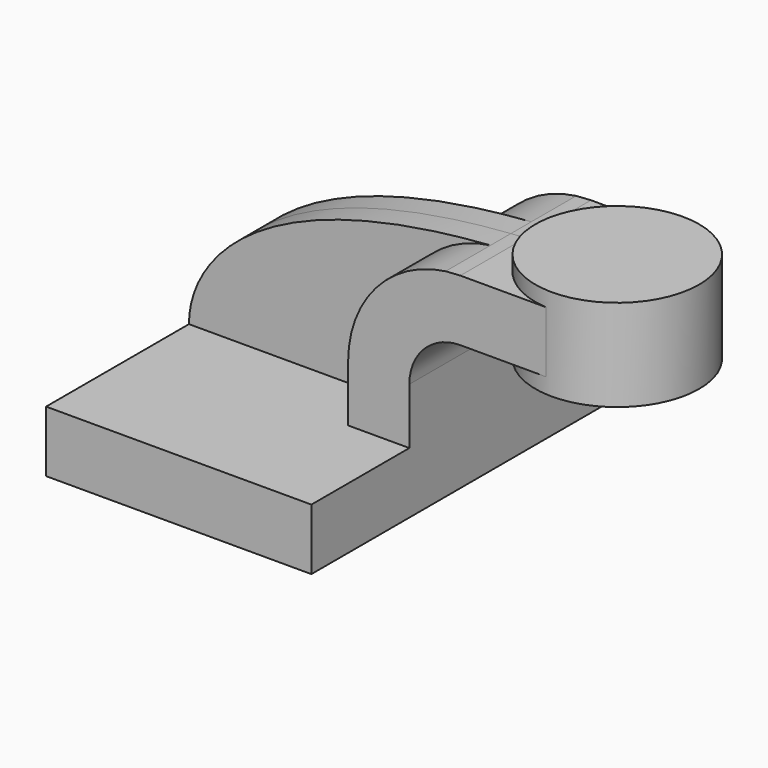
from build123d import *

# Parameters (mm, degrees)
F1_DEPTH = 63.5
F0_W     = 25.3298562567
F0_H     = 19.05
F2_DEPTH = 25.4
F3_DEPTH = 7.9375


with BuildPart() as f1:
    # F0 (on Front) → F1 (new body, symmetric)
    with BuildSketch(Plane.XZ):
        Polygon((-41.275, 9.525), (-41.275, -9.525), (41.275, -9.525), (41.275, 9.525), (22.225, 9.525), align=None)
    extrude(amount=F1_DEPTH, both=True)

    # F0 (on Front) → F2 (join, symmetric)
    with BuildSketch(Plane.XZ):
        with BuildLine():
            Line((22.225, 9.525), (41.275, 9.525))
            Line((41.275, 9.525), (41.275, 27.0002))
            ThreePointArc((41.275, 27.0002), (45.9246798487, 38.2255201513), (57.15, 42.8752))
            Line((57.15, 42.8752), (60.325, 42.8752))
            Line((60.325, 42.8752), (60.325, 61.9252))
            Line((60.325, 61.9252), (57.15, 61.9252))
            add(Edge.make_bspline(
                [(52.5566804935, 61.6218267803), (54.0650417221, 61.7326720686), (55.596048457, 61.833893026), (57.15, 61.9252)],
                knots=[109.2974079023, 109.2974079023, 109.2974079023, 109.2974079023, 111.5045361635, 111.5045361635, 111.5045361635, 111.5045361635], degree=3))
            ThreePointArc((52.5566804935, 61.6218267803), (30.8804614738, 50.0146947939), (22.225, 27.0002))
            Line((22.225, 27.0002), (22.225, 9.525))
        make_face()
        with Locations((72.9899281284, 52.4002)):
            Rectangle(F0_W, F0_H)
    extrude(amount=F2_DEPTH, both=True)

    # F0 (on Front) → F3 (join, symmetric)
    with BuildSketch(Plane.XZ):
        with BuildLine():
            add(Edge.make_bspline(
                [(-41.275, 9.525), (-41.2995623579, 27.0424108455), (-22.1376521166, 56.1327471898), (52.5566804935, 61.6218267803)],
                knots=[0, 0, 0, 0, 109.2974079023, 109.2974079023, 109.2974079023, 109.2974079023], degree=3))
            Line((-41.275, 9.525), (22.225, 9.525))
            Line((22.225, 9.525), (22.225, 27.0002))
            ThreePointArc((22.225, 27.0002), (30.8804614738, 50.0146947939), (52.5566804935, 61.6218267803))
        make_face()
    extrude(amount=F3_DEPTH, both=True)

    # F0 (on Front) → F4 (revolve)
    with BuildSketch(Plane.XZ):
        Polygon((85.6548562567, 66.675), (85.6548562567, 61.9252), (85.6548562567, 42.8752), (85.6548562567, 38.1), (111.125, 38.1), (111.125, 66.675), align=None)
    revolve(axis=Axis((85.6548562567, 0, 52.3875), (0, 0, 1)))


solid = f1.part
